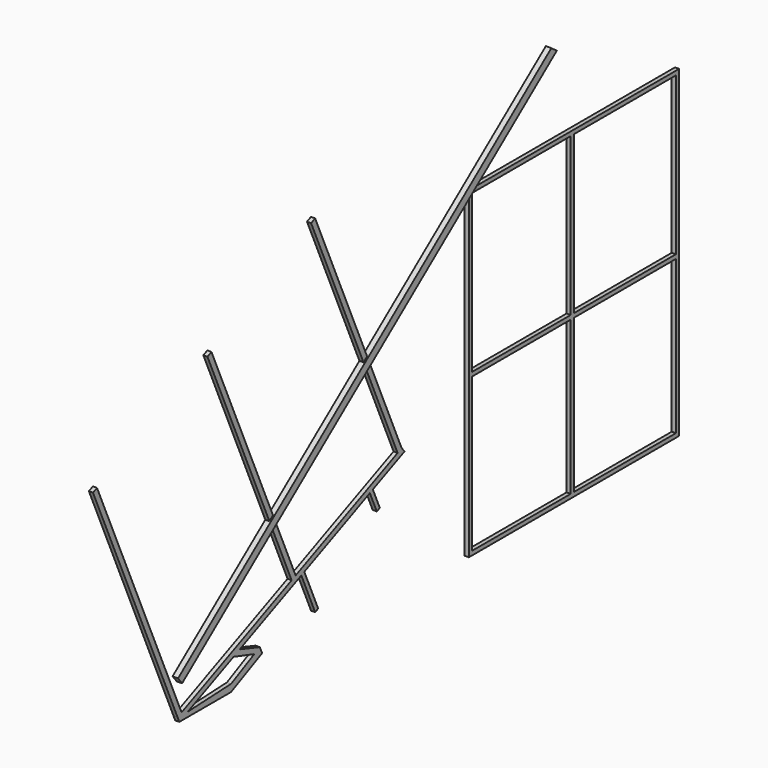
from build123d import *

# Parameters (mm, degrees)
F0_W      = 2440
F0_H      = 3000
F0_W_2    = 2363.8
F0_H_2    = 2923.8
F1_DEPTH  = 38.1
F2_W      = 38.1
F2_H      = 3000
F3_DEPTH  = 38.1
F4_W      = 2440
F4_H      = 38.1
F5_DEPTH  = 38.1
F7_DEPTH  = 38.1
F9_DEPTH  = 38.1
F10_DEPTH = 38.1
F11_W     = 38.1
F11_H     = 38.1
F12_DEPTH = 200
F13_W     = 38.1
F13_H     = 38.1
F14_DEPTH = 200
F16_DEPTH = 50.8


# Not quite as in the source:
# - a feature names something its author has since deleted; it is built from what else it names


with BuildPart() as f1:
    # F0 (on Right) → F1 (new body)
    with BuildSketch(Plane.YZ):
        with Locations((4653.3635152385, 965.0668048064)):
            Rectangle(F0_W, F0_H)
        with Locations((4653.3635152385, 965.0668048064)):
            Rectangle(F0_W_2, F0_H_2, mode=Mode.SUBTRACT)
    extrude(amount=F1_DEPTH)

    # F2 (on face) → F3 (join)
    with BuildSketch(Plane.YZ.offset(38.1)):
        with Locations((4634.3135152385, 965.0668048064)):
            Rectangle(F2_W, F2_H)
    extrude(amount=-F3_DEPTH)

    # F4 (on face) → F5 (join)
    with BuildSketch(Plane.YZ.offset(38.1)):
        with Locations((4653.3635152385, 946.0168048064)):
            Rectangle(F4_W, F4_H)
    extrude(amount=-F5_DEPTH)


with BuildPart() as f7:
    # F6 (on Right) → F7 (new body)
    with BuildSketch(Plane.YZ):
        Polygon((74.091359973, -514.4183039665), (2689.3315110135, 634.3592099591), (2653.8618600197, 674.2636581614), (2607.3512244074, 653.8332696449), (1423.7013476008, 133.8999999239), (1377.1907119885, 113.4696114073), (100.1716070687, -447.4772798376), (109.1459151908, -467.9076683542), align=None)
        Polygon((53.6609714564, -467.9076683542), (74.091359973, -514.4183039665), (109.1459151908, -467.9076683542), (100.1716070687, -447.4772798376), align=None)
        Polygon((2607.3512244074, 653.8332696449), (2653.8618600197, 674.2636581614), (1649.6657982272, 2960.358074601), (1603.1551626149, 2939.9276860845), align=None)
        Polygon((-927.6411541415, 1766.0677429467), (53.6609714564, -467.9076683542), (100.1716070687, -447.4772798376), (-881.1305185292, 1786.4981314632), align=None)
        Polygon((1377.1907119885, 113.4696114073), (1423.7013476008, 133.8999999239), (446.9199455077, 2357.5837947211), (400.4093098953, 2337.1534062045), align=None)
    extrude(amount=F7_DEPTH)

    # F8 (on face) → F9 (join)
    with BuildSketch(Plane.YZ.offset(38.1)):
        Polygon((943.2376147162, -313.9598791054), (1035.5579565697, -343.1235301269), (1006.796002388, -282.4299931526), align=None)
        Polygon((173.1557213069, -470.9030227077), (74.091359973, -514.4183039665), (674.091359973, -514.4183039665), (674.091359973, -447.4772798376), align=None)
        Polygon((674.091359973, -447.4772798376), (674.091359973, -514.4183039665), (1035.5579565697, -343.1235301269), (943.2376147162, -313.9598791054), align=None)
    extrude(amount=-F9_DEPTH)

    # F8 (on face) → F10 (join)
    with BuildSketch(Plane.YZ.offset(38.1)):
        Polygon((674.091359973, -447.4772798376), (674.091359973, -514.4183039665), (1035.5579565697, -343.1235301269), (943.2376147162, -313.9598791054), align=None)
        Polygon((943.2376147162, -313.9598791054), (1035.5579565697, -343.1235301269), (1006.796002388, -282.4299931526), align=None)
        Polygon((703.1224470539, -238.1083948703), (943.2376147162, -313.9598791054), (1006.796002388, -282.4299931526), (775.7308186411, -206.2142437466), align=None)
    extrude(amount=-F10_DEPTH)

    # F11 (on face) → F12 (join)
    with BuildSketch(Plane(origin=(0, 201.4003034253, -458.4962306145), x_dir=(1, 0, 0), z_dir=(0, 0.4021730023, -0.9155636932))):
        with Locations((19.05, -1426.0808250427)):
            Rectangle(F11_W, F11_H)
        with Locations((19.05, -2294.8585769653)):
            Rectangle(F11_W, F11_H)
    extrude(amount=F12_DEPTH)

    # F13 (on face) → F14 (join)
    with BuildSketch(Plane(origin=(0, 281.8349038841, -641.6089692457), x_dir=(1, 0, 0), z_dir=(0, 0.4021730023, -0.9155636932))):
        with Locations((19.05, -1426.0808250427)):
            Rectangle(F13_W, F13_H)
    extrude(amount=F14_DEPTH)


with BuildPart() as f16:
    # F15 (on Right) → F16 (new body)
    with BuildSketch(Plane.YZ):
        Polygon((90.4242247343, -201.7892897129), (4438.0540736265, 3200.8221953591), (4374.6806999502, 3247.9864848224), (43.4605203704, -141.7822028613), align=None)
    extrude(amount=F16_DEPTH)


solid = Compound([f1.part, f7.part, f16.part])
